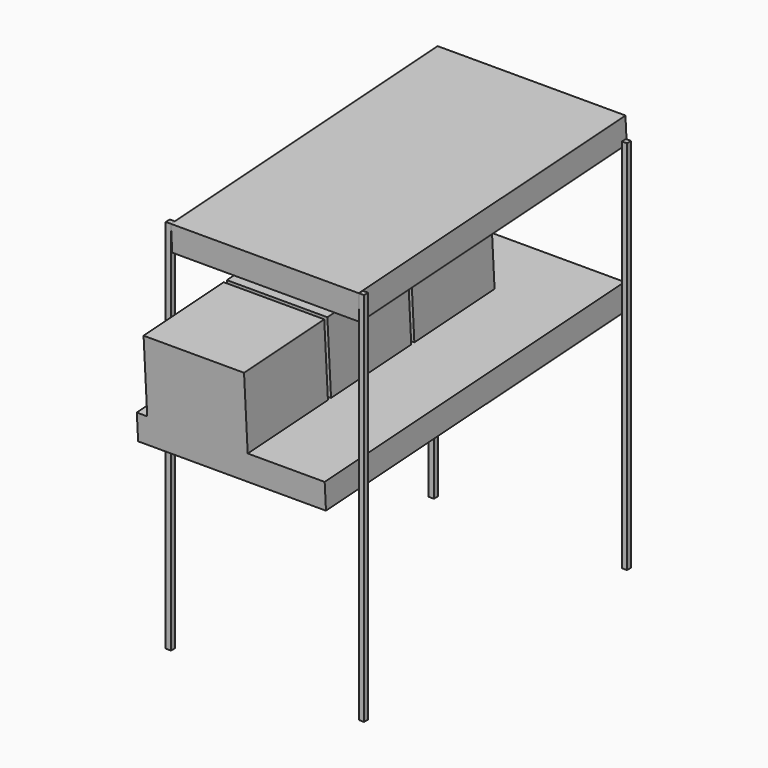
from build123d import *

# Parameters (mm, degrees)
F2_W      = 12.7
F2_H      = 12.7
F3_DEPTH  = 914.4
F6_W      = 457.2
F6_H      = 914.4
F7_DEPTH  = 63.5
F10_W     = 457.2
F10_H     = 812.8
F11_DEPTH = 63.5
F12_W     = 244.475
F12_H     = 244.475
F13_DEPTH = 177.8


# Not quite as in the source:
# - the program builds the solid bodies; features that only make, move or delete a surface that nothing else refers to are left out


with BuildPart() as f3:
    # F2 (on Top) → F3 (new body, through all)
    with BuildSketch(Plane.XY):
        with Locations((-234.95, 6.35)):
            Rectangle(F2_W, F2_H)
    extrude(amount=F3_DEPTH)


with BuildPart() as f3b:
    # F2 (on Top) → F3, piece 2 (new body, through all)
    with BuildSketch(Plane.XY):
        with Locations((234.95, 6.35)):
            Rectangle(F2_W, F2_H)
    extrude(amount=F3_DEPTH)


with BuildPart() as f3c:
    # F2 (on Top) → F3, piece 3 (new body, through all)
    with BuildSketch(Plane.XY):
        with Locations((234.95, 806.45)):
            Rectangle(F2_W, F2_H)
    extrude(amount=F3_DEPTH)


with BuildPart() as f3d:
    # F2 (on Top) → F3, piece 4 (new body, through all)
    with BuildSketch(Plane.XY):
        with Locations((-234.95, 806.45)):
            Rectangle(F2_W, F2_H)
    extrude(amount=F3_DEPTH)


with BuildPart() as f7:
    # F6 (on face) → F7 (new body)
    with BuildSketch(Plane(origin=(0, -35.0181054579, 556.5968475473), x_dir=(1, 0, 0), z_dir=(0, 0.0627905195, -0.9980267284))):
        with Locations((0, -388.3167412758)):
            Rectangle(F6_W, F6_H)
    extrude(amount=F7_DEPTH)

    # F12 (on face) → F13 (join)
    with BuildSketch(Plane(origin=(0, -35.0181054579, 556.5968475473), x_dir=(1, 0, 0), z_dir=(0, 0.0627905195, -0.9980267284))):
        with Locations((-80.9625, -53.3542412758)):
            Rectangle(F12_W, F12_H)
        with Locations((-80.9625, -307.3542412758)):
            Rectangle(F12_W, F12_H)
        with Locations((-80.9625, -561.3542412758)):
            Rectangle(F12_W, F12_H)
    extrude(amount=-F13_DEPTH)


with BuildPart() as f11:
    # F10 (on face) → F11 (new body)
    with BuildSketch(Plane(origin=(0, -57.3023543856, 910.794841441), x_dir=(1, 0, 0), z_dir=(0, 0.0627905195, -0.9980267284))):
        with Locations((0, -463.8156510576)):
            Rectangle(F10_W, F10_H)
    extrude(amount=F11_DEPTH)


solid = Compound([f3.part, f3b.part, f3c.part, f3d.part, f7.part, f11.part])
